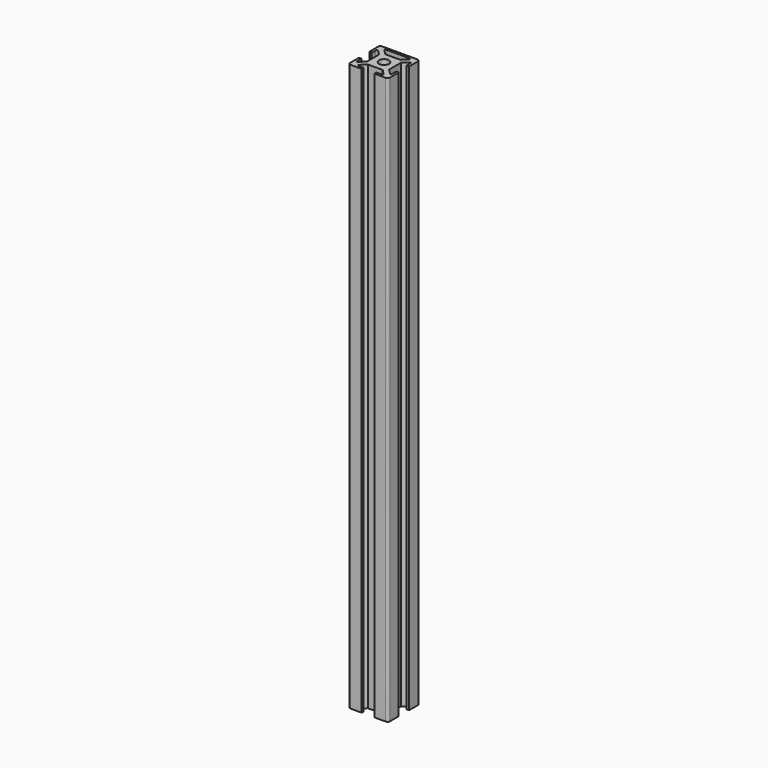
from build123d import *

# Parameters (mm, degrees)
F0_W        = 25.4
F0_H        = 25.4
F1_DEPTH    = 455.93
F3_DEPTH    = 455.93
F4_R        = 3.175
F5_DEPTH    = 455.93
F6_T1_DEPTH = 463.8675
F7_T1_DEPTH = 455.93
F8_W        = 8.2098719395
F8_H        = 1.5875
F9_DEPTH    = 455.93
F10_DEPTH   = 93.98


# Not quite as in the source:
# - a fillet or chamfer that OpenCascade refuses, or shapes differently, is made with other operations: its cross-section is extruded or revolved along the edge and cut away or added


with BuildPart() as f1:
    # F0 (on Top) → F1 (new body)
    with BuildSketch(Plane.XY):
        Rectangle(F0_W, F0_H)
    extrude(amount=F1_DEPTH)

    # F2 (on face) → F3 (cut)
    with BuildSketch(Plane.XY.offset(455.93)):
        Polygon((-7.0075640303, -4.7625), (-7.0075640303, 4.7625), (-11.1125, 8.8674359697), (-11.1125, 4.1049359697), (-12.7, 4.1049359697), (-12.7, -4.1049359697), (-11.1125, -4.1049359697), (-11.1125, -8.8674359697), align=None)
        Polygon((4.1049359697, 12.7), (-4.1049359697, 12.7), (-4.1049359697, 11.1125), (-8.8674359697, 11.1125), (-4.7625, 7.0075640303), (4.7625, 7.0075640303), (8.8674359697, 11.1125), (4.1049359697, 11.1125), align=None)
        Polygon((12.7, -4.1049359697), (12.7, 4.1049359697), (11.1125, 4.1049359697), (11.1125, 8.8674359697), (7.0075640303, 4.7625), (7.0075640303, -4.7625), (11.1125, -8.8674359697), (11.1125, -4.1049359697), align=None)
        Polygon((-4.1049359697, -11.1125), (-4.1049359697, -12.7), (4.1049359697, -12.7), (4.1049359697, -11.1125), (8.8674359697, -11.1125), (4.7625, -7.0075640303), (-4.7625, -7.0075640303), (-8.8674359697, -11.1125), align=None)
    extrude(amount=-F3_DEPTH, mode=Mode.SUBTRACT)

    # F4 (on face) → F5 (cut)
    with BuildSketch(Plane.XY.offset(455.93)):
        Circle(F4_R)
    extrude(amount=-F5_DEPTH, mode=Mode.SUBTRACT)

    # F6: fillet of radius 1.5875 on 4 edges, made by hand

    # F6_s2 → F6_t1 (cut)
    with BuildSketch(Plane.XY.offset(-3.96875)):
        with BuildLine():
            add(Edge.make_bspline(
                [(-12.7, 11.1125), (-12.7, 12.7), (-11.1125, 12.7)],
                knots=[0, 0, 0, 1, 1, 1], degree=2, weights=[1, 1, 1]))
            Line((-11.1125, 12.7), (-12.7, 12.7))
            Line((-12.7, 12.7), (-12.7, 11.1125))
        make_face()
        with BuildLine():
            add(Edge.make_bspline(
                [(12.7, 11.1125), (12.7, 12.7), (11.1125, 12.7)],
                knots=[0, 0, 0, 1, 1, 1], degree=2, weights=[1, 1, 1]))
            Line((11.1125, 12.7), (12.7, 12.7))
            Line((12.7, 12.7), (12.7, 11.1125))
        make_face()
        with BuildLine():
            add(Edge.make_bspline(
                [(12.7, -11.1125), (12.7, -12.7), (11.1125, -12.7)],
                knots=[0, 0, 0, 1, 1, 1], degree=2, weights=[1, 1, 1]))
            Line((11.1125, -12.7), (12.7, -12.7))
            Line((12.7, -12.7), (12.7, -11.1125))
        make_face()
        with BuildLine():
            add(Edge.make_bspline(
                [(-11.1125, -12.7), (-12.7, -12.7), (-12.7, -11.1125)],
                knots=[0, 0, 0, 1, 1, 1], degree=2, weights=[1, 1, 1]))
            Line((-12.7, -11.1125), (-12.7, -12.7))
            Line((-12.7, -12.7), (-11.1125, -12.7))
        make_face()
    extrude(amount=F6_T1_DEPTH, mode=Mode.SUBTRACT)

    # F7: fillet of radius 0.79375 on 8 edges, made by hand

    # F7_s2 → F7_t1 (join)
    with BuildSketch(Plane.XY):
        with BuildLine():
            add(Edge.make_bspline(
                [(-9.7574839924, 7.5124199622), (-11.1125, 8.8674359697), (-11.1125, 6.9511539546)],
                knots=[0, 0, 0, 1, 1, 1], degree=2, weights=[1, 1, 1]))
            Line((-11.1125, 6.9511539546), (-11.1125, 8.8674359697))
            Line((-11.1125, 8.8674359697), (-9.7574839924, 7.5124199622))
        make_face()
        with BuildLine():
            add(Edge.make_bspline(
                [(11.1125, 6.9511539546), (11.1125, 8.8674359697), (9.7574839924, 7.5124199622)],
                knots=[0, 0, 0, 1, 1, 1], degree=2, weights=[1, 1, 1]))
            Line((9.7574839924, 7.5124199622), (11.1125, 8.8674359697))
            Line((11.1125, 8.8674359697), (11.1125, 6.9511539546))
        make_face()
        with BuildLine():
            add(Edge.make_bspline(
                [(9.7574839924, -7.5124199622), (11.1125, -8.8674359697), (11.1125, -6.9511539546)],
                knots=[0, 0, 0, 1, 1, 1], degree=2, weights=[1, 1, 1]))
            Line((11.1125, -6.9511539546), (11.1125, -8.8674359697))
            Line((11.1125, -8.8674359697), (9.7574839924, -7.5124199622))
        make_face()
        with BuildLine():
            add(Edge.make_bspline(
                [(-11.1125, -6.9511539546), (-11.1125, -8.8674359697), (-9.7574839924, -7.5124199622)],
                knots=[0, 0, 0, 1, 1, 1], degree=2, weights=[1, 1, 1]))
            Line((-9.7574839924, -7.5124199622), (-11.1125, -8.8674359697))
            Line((-11.1125, -8.8674359697), (-11.1125, -6.9511539546))
        make_face()
        with BuildLine():
            add(Edge.make_bspline(
                [(-7.5124199622, -9.7574839924), (-8.8674359697, -11.1125), (-6.9511539546, -11.1125)],
                knots=[0, 0, 0, 1, 1, 1], degree=2, weights=[1, 1, 1]))
            Line((-6.9511539546, -11.1125), (-8.8674359697, -11.1125))
            Line((-8.8674359697, -11.1125), (-7.5124199622, -9.7574839924))
        make_face()
        with BuildLine():
            add(Edge.make_bspline(
                [(6.9511539546, -11.1125), (8.8674359697, -11.1125), (7.5124199622, -9.7574839924)],
                knots=[0, 0, 0, 1, 1, 1], degree=2, weights=[1, 1, 1]))
            Line((7.5124199622, -9.7574839924), (8.8674359697, -11.1125))
            Line((8.8674359697, -11.1125), (6.9511539546, -11.1125))
        make_face()
        with BuildLine():
            add(Edge.make_bspline(
                [(7.5124199622, 9.7574839924), (8.8674359697, 11.1125), (6.9511539546, 11.1125)],
                knots=[0, 0, 0, 1, 1, 1], degree=2, weights=[1, 1, 1]))
            Line((6.9511539546, 11.1125), (8.8674359697, 11.1125))
            Line((8.8674359697, 11.1125), (7.5124199622, 9.7574839924))
        make_face()
        with BuildLine():
            add(Edge.make_bspline(
                [(-6.9511539546, 11.1125), (-8.8674359697, 11.1125), (-7.5124199622, 9.7574839924)],
                knots=[0, 0, 0, 1, 1, 1], degree=2, weights=[1, 1, 1]))
            Line((-7.5124199622, 9.7574839924), (-8.8674359697, 11.1125))
            Line((-8.8674359697, 11.1125), (-6.9511539546, 11.1125))
        make_face()
    extrude(amount=F7_T1_DEPTH)

    # F8 (on face) → F9 (join)
    with BuildSketch(Plane.XY.offset(455.93)):
        with Locations((0, 11.90625)):
            Rectangle(F8_W, F8_H)
    extrude(amount=-F9_DEPTH)

    # F10 (cut): a face of the model
    f10_faces = [f1.faces().sort_by_distance(p)[0] for p in [
        (4.4641462174, -11.90625, 455.93),
    ]]
    extrude(f10_faces, amount=-F10_DEPTH, mode=Mode.SUBTRACT)


solid = f1.part
